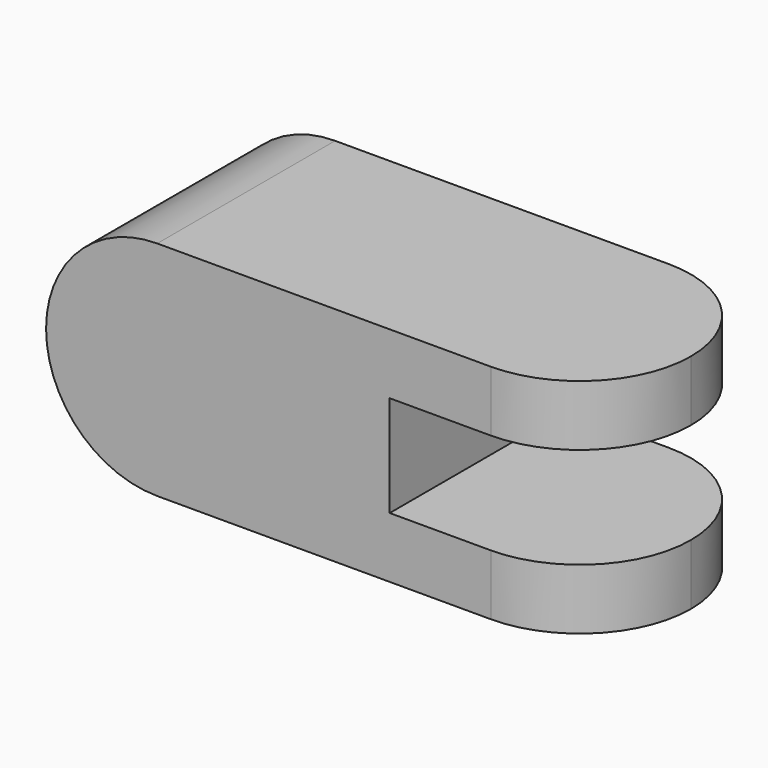
from build123d import *

# Parameters (mm, degrees)
F0_W          = 139.7
F0_H          = 55.88
F1_DEPTH      = 55.88
F2_R          = 27.93999
F3_W          = 53.34
F3_H          = 25.4
F4_DEPTH      = 6.9680017111
F4_DEPTH_BACK = 48.9139982889


# Not quite as in the source:
# - a fillet or chamfer is up to 0.001 mm smaller than in the source, because OpenCascade refuses the exact size


with BuildPart() as f1:
    # F0 (on Top) → F1 (new body)
    with BuildSketch(Plane.XY):
        with Locations((19.5538900733, -20.9729982889)):
            Rectangle(F0_W, F0_H)
    extrude(amount=F1_DEPTH)

    # F2 (radius 27.94 in the source; OpenCascade refuses exactly that, so slightly less here)
    f2_edges = [f1.edges().sort_by_distance(p)[0] for p in [
        (-50.29611, -20.972998, 0),
        (-50.29611, -20.972998, 55.88),
        (89.40389, -48.912998, 27.94),
        (89.40389, 6.967002, 27.94),
    ]]
    fillet(f2_edges, radius=F2_R)

    # F3 (on Front) → F4 (cut, two sides)
    with BuildSketch(Plane.XZ) as f4_sk:
        with Locations((62.7338900733, 27.94)):
            Rectangle(F3_W, F3_H)
    extrude(amount=-F4_DEPTH, mode=Mode.SUBTRACT)
    extrude(f4_sk.sketch, amount=F4_DEPTH_BACK, mode=Mode.SUBTRACT)


solid = f1.part
